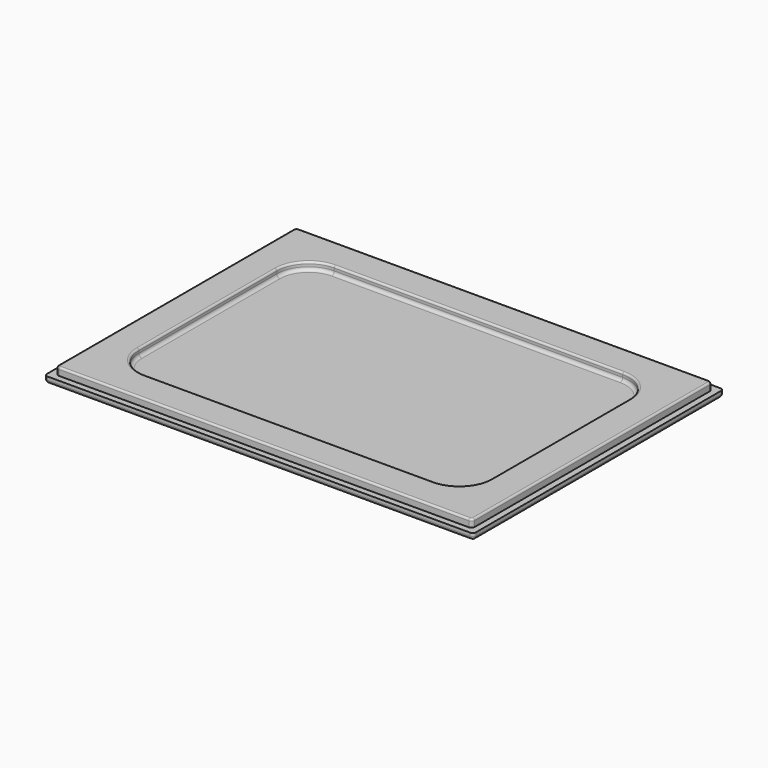
from build123d import *

# Parameters (mm, degrees)
F0_W         = 67.2
F0_H         = 49
F1_DEPTH     = 1
F2_DEPTH     = 2.2
F3_R         = 0.5
F4_R         = 0.3
F5_S2_W      = 0.5
F5_S2_H      = 0.5
F5_T3_DEPTH  = 0.5
F5_T8_ANGLE  = 90
F5_S10_W     = 0.5
F5_S10_H     = 0.5
F5_T11_DEPTH = 0.5
F5_T16_ANGLE = 90
F5_S18_W     = 0.5
F5_S18_H     = 0.5
F5_T19_DEPTH = 0.5
F5_T24_ANGLE = 90
F5_S26_W     = 0.5
F5_S26_H     = 0.5
F5_T27_DEPTH = 0.5
F5_T32_ANGLE = 90
F5_T35_DEPTH = 1.2
F5_T38_DEPTH = 1.75
F5_T41_DEPTH = 1.2
F5_T44_DEPTH = 1.75
F5_T47_DEPTH = 1.2
F5_T50_DEPTH = 1.75
F5_T53_DEPTH = 1.2
F5_T56_DEPTH = 1.75
F6_R         = 0.5


# Not quite as in the source:
# - a fillet or chamfer that OpenCascade refuses, or shapes differently, is made with other operations: its cross-section is extruded or revolved along the edge and cut away or added


with BuildPart() as f1:
    # F0 (on Top) → F1 (new body)
    with BuildSketch(Plane.XY):
        with Locations((8.3761618346, 4.5501037389)):
            Rectangle(F0_W, F0_H)
        Polygon((-24.2238381654, 20.0501037389), (-24.2238381654, 28.0501037389), (-16.2238381654, 28.0501037389), (32.9761618346, 28.0501037389), (40.9761618346, 28.0501037389), (40.9761618346, 20.0501037389), (40.9761618346, -10.9498962611), (40.9761618346, -18.9498962611), (32.9761618346, -18.9498962611), (-16.2238381654, -18.9498962611), (-24.2238381654, -18.9498962611), (-24.2238381654, -10.9498962611), align=None, mode=Mode.SUBTRACT)
        Polygon((-16.2238381654, 28.0501037389), (-24.2238381654, 28.0501037389), (-24.2238381654, 20.0501037389), (-24.2238381654, -10.9498962611), (-24.2238381654, -18.9498962611), (-16.2238381654, -18.9498962611), (32.9761618346, -18.9498962611), (40.9761618346, -18.9498962611), (40.9761618346, -10.9498962611), (40.9761618346, 20.0501037389), (40.9761618346, 28.0501037389), (32.9761618346, 28.0501037389), align=None)
        with BuildLine():
            ThreePointArc((-19.2238390446, 18.0501037389), (-17.7593729505, 21.5856376448), (-14.2238390446, 23.0501037389))
            Line((-14.2238390446, 23.0501037389), (30.9761627138, 23.0501037389))
            ThreePointArc((30.9761627138, 23.0501037389), (34.5116966197, 21.5856376448), (35.9761627138, 18.0501037389))
            Line((35.9761627138, 18.0501037389), (35.9761627138, -8.9498971403))
            ThreePointArc((35.9761627138, -8.9498971403), (34.5116966197, -12.4854310462), (30.9761627138, -13.9498971403))
            Line((30.9761627138, -13.9498971403), (-14.2238390446, -13.9498971403))
            ThreePointArc((-14.2238390446, -13.9498971403), (-17.7593729505, -12.4854310462), (-19.2238390446, -8.9498971403))
            Line((-19.2238390446, -8.9498971403), (-19.2238390446, 18.0501037389))
        make_face(mode=Mode.SUBTRACT)
        with BuildLine():
            Line((30.9761627138, 23.0501037389), (-14.2238390446, 23.0501037389))
            ThreePointArc((-14.2238390446, 23.0501037389), (-17.7593729505, 21.5856376448), (-19.2238390446, 18.0501037389))
            Line((-19.2238390446, 18.0501037389), (-19.2238390446, -8.9498971403))
            ThreePointArc((-19.2238390446, -8.9498971403), (-17.7593729505, -12.4854310462), (-14.2238390446, -13.9498971403))
            Line((-14.2238390446, -13.9498971403), (30.9761627138, -13.9498971403))
            ThreePointArc((30.9761627138, -13.9498971403), (34.5116966197, -12.4854310462), (35.9761627138, -8.9498971403))
            Line((35.9761627138, -8.9498971403), (35.9761627138, 18.0501037389))
            ThreePointArc((35.9761627138, 18.0501037389), (34.5116966197, 21.5856376448), (30.9761627138, 23.0501037389))
        make_face()
    extrude(amount=F1_DEPTH)

    # F0 (on Top) → F2 (join)
    with BuildSketch(Plane.XY):
        Polygon((-16.2238381654, 28.0501037389), (-24.2238381654, 28.0501037389), (-24.2238381654, 20.0501037389), (-24.2238381654, -10.9498962611), (-24.2238381654, -18.9498962611), (-16.2238381654, -18.9498962611), (32.9761618346, -18.9498962611), (40.9761618346, -18.9498962611), (40.9761618346, -10.9498962611), (40.9761618346, 20.0501037389), (40.9761618346, 28.0501037389), (32.9761618346, 28.0501037389), align=None)
        with BuildLine():
            ThreePointArc((-19.2238390446, 18.0501037389), (-17.7593729505, 21.5856376448), (-14.2238390446, 23.0501037389))
            Line((-14.2238390446, 23.0501037389), (30.9761627138, 23.0501037389))
            ThreePointArc((30.9761627138, 23.0501037389), (34.5116966197, 21.5856376448), (35.9761627138, 18.0501037389))
            Line((35.9761627138, 18.0501037389), (35.9761627138, -8.9498971403))
            ThreePointArc((35.9761627138, -8.9498971403), (34.5116966197, -12.4854310462), (30.9761627138, -13.9498971403))
            Line((30.9761627138, -13.9498971403), (-14.2238390446, -13.9498971403))
            ThreePointArc((-14.2238390446, -13.9498971403), (-17.7593729505, -12.4854310462), (-19.2238390446, -8.9498971403))
            Line((-19.2238390446, -8.9498971403), (-19.2238390446, 18.0501037389))
        make_face(mode=Mode.SUBTRACT)
    extrude(amount=F2_DEPTH)

    # F3
    f3_edges = [f1.edges().sort_by_distance(p)[0] for p in [
        (41.976162, 4.550104, 0),
        (8.376162, 29.050104, 0),
        (-25.223838, 4.550104, 0),
        (8.376162, -19.949896, 0),
    ]]
    fillet(f3_edges, radius=F3_R)

    # F4
    f4_edges = [f1.edges().sort_by_distance(p)[0] for p in [
        (8.376162, 28.050104, 2.2),
        (-24.223838, 4.550104, 2.2),
        (8.376162, -18.949896, 2.2),
        (40.976162, 4.550104, 2.2),
        (-19.223839, 4.550103, 2.2),
        (-17.759373, 21.585638, 2.2),
        (8.376162, 23.050104, 2.2),
        (34.511697, 21.585638, 2.2),
        (35.976163, 4.550103, 2.2),
        (34.511697, -12.485431, 2.2),
        (8.376162, -13.949897, 2.2),
        (-17.759373, -12.485431, 2.2),
    ]]
    fillet(f4_edges, radius=F4_R)

    # F5: fillet of radius 0.5 on 8 edges, made by hand


with BuildPart() as f5_tool1:
    # F5_s2 → F5_t3 (new body)
    with BuildSketch(Plane.XZ.offset(-28.5501037389)):
        with Locations((-24.9738381654, 0.25)):
            Rectangle(F5_S2_W, F5_S2_H)
    extrude(amount=-F5_T3_DEPTH)

    # F5_s4 → F5_t5 (revolve, cut)
    with BuildSketch(Plane(origin=(-24.7238381654, 28.5501037389, 0.5), x_dir=(0.7071067812, 0, 0.7071067812), z_dir=(-0.7071067812, 0, 0.7071067812))):
        with BuildLine():
            ThreePointArc((0, -0.5), (0.5, 0), (0, 0.5))
            Line((0, 0.5), (0, -0.5))
        make_face()
    revolve(axis=Axis((-24.7238381654, 28.5501037389, 0.5), (0, 1, 0)), mode=Mode.SUBTRACT)


with BuildPart() as f5_tool6:
    # F5_s7 → F5_t8 (revolve)
    with BuildSketch(Plane.YZ.offset(-23.7238381654)):
        with BuildLine():
            ThreePointArc((27.7501037389, 2.2), (27.9622357733, 2.1121320344), (28.0501037389, 1.9))
            Line((28.0501037389, 1.9), (28.0501037389, 2.2))
            Line((28.0501037389, 2.2), (27.7501037389, 2.2))
        make_face()
    revolve(axis=Axis((-23.7238381654, 27.5501037389, 2.2), (0, 0, 1)), revolution_arc=F5_T8_ANGLE)


with BuildPart() as f5_tool9:
    # F5_s10 → F5_t11 (new body)
    with BuildSketch(Plane.XZ.offset(19.4498962611)):
        with Locations((-24.9738381654, 0.25)):
            Rectangle(F5_S10_W, F5_S10_H)
    extrude(amount=F5_T11_DEPTH)

    # F5_s12 → F5_t13 (revolve, cut)
    with BuildSketch(Plane(origin=(-24.7238381654, -19.4498962611, 0.5), x_dir=(0.7071067812, 0, 0.7071067812), z_dir=(0.7071067812, 0, -0.7071067812))):
        with BuildLine():
            ThreePointArc((0, -0.5), (0.5, 0), (0, 0.5))
            Line((0, 0.5), (0, -0.5))
        make_face()
    revolve(axis=Axis((-24.7238381654, -19.4498962611, 0.5), (0, -1, 0)), mode=Mode.SUBTRACT)


with BuildPart() as f5_tool14:
    # F5_s15 → F5_t16 (revolve)
    with BuildSketch(Plane.XZ.offset(18.4498962611)):
        with BuildLine():
            ThreePointArc((-23.9238381654, 2.2), (-24.1359701998, 2.1121320344), (-24.2238381654, 1.9))
            Line((-24.2238381654, 1.9), (-24.2238381654, 2.2))
            Line((-24.2238381654, 2.2), (-23.9238381654, 2.2))
        make_face()
    revolve(axis=Axis((-23.7238381654, -18.4498962611, 2.2), (0, 0, 1)), revolution_arc=F5_T16_ANGLE)


with BuildPart() as f5_tool17:
    # F5_s18 → F5_t19 (new body)
    with BuildSketch(Plane.YZ.offset(41.4761618346)):
        with Locations((-19.6998962611, 0.25)):
            Rectangle(F5_S18_W, F5_S18_H)
    extrude(amount=F5_T19_DEPTH)

    # F5_s20 → F5_t21 (revolve, cut)
    with BuildSketch(Plane(origin=(41.4761618346, -19.4498962611, 0.5), x_dir=(0, 0.7071067812, 0.7071067812), z_dir=(0, 0.7071067812, -0.7071067812))):
        with BuildLine():
            ThreePointArc((0, -0.5), (0.5, 0), (0, 0.5))
            Line((0, 0.5), (0, -0.5))
        make_face()
    revolve(axis=Axis((41.4761618346, -19.4498962611, 0.5), (1, 0, 0)), mode=Mode.SUBTRACT)


with BuildPart() as f5_tool22:
    # F5_s23 → F5_t24 (revolve)
    with BuildSketch(Plane.YZ.offset(40.4761618346)):
        with BuildLine():
            ThreePointArc((-18.6498962611, 2.2), (-18.8620282955, 2.1121320344), (-18.9498962611, 1.9))
            Line((-18.9498962611, 1.9), (-18.9498962611, 2.2))
            Line((-18.9498962611, 2.2), (-18.6498962611, 2.2))
        make_face()
    revolve(axis=Axis((40.4761618346, -18.4498962611, 2.2), (0, 0, 1)), revolution_arc=F5_T24_ANGLE)


with BuildPart() as f5_tool25:
    # F5_s26 → F5_t27 (new body)
    with BuildSketch(Plane.YZ.offset(41.4761618346)):
        with Locations((28.8001037389, 0.25)):
            Rectangle(F5_S26_W, F5_S26_H)
    extrude(amount=F5_T27_DEPTH)

    # F5_s28 → F5_t29 (revolve, cut)
    with BuildSketch(Plane(origin=(41.4761618346, 28.5501037389, 0.5), x_dir=(0, -0.7071067812, 0.7071067812), z_dir=(0, 0.7071067812, 0.7071067812))):
        with BuildLine():
            ThreePointArc((0, -0.5), (0.5, 0), (0, 0.5))
            Line((0, 0.5), (0, -0.5))
        make_face()
    revolve(axis=Axis((41.4761618346, 28.5501037389, 0.5), (1, 0, 0)), mode=Mode.SUBTRACT)


with BuildPart() as f5_tool30:
    # F5_s31 → F5_t32 (revolve)
    with BuildSketch(Plane.XZ.offset(-27.5501037389)):
        with BuildLine():
            ThreePointArc((40.6761618346, 2.2), (40.888293869, 2.1121320344), (40.9761618346, 1.9))
            Line((40.9761618346, 1.9), (40.9761618346, 2.2))
            Line((40.9761618346, 2.2), (40.6761618346, 2.2))
        make_face()
    revolve(axis=Axis((40.4761618346, 27.5501037389, 2.2), (0, 0, 1)), revolution_arc=F5_T32_ANGLE)


with BuildPart() as f5_tool33:
    # F5_s34 → F5_t35 (new body)
    with BuildSketch(Plane.XY.offset(1)):
        with BuildLine():
            ThreePointArc((40.4761618346, 28.0501037389), (40.8297152252, 27.9036571295), (40.9761618346, 27.5501037389))
            Line((40.9761618346, 27.5501037389), (40.9761618346, 28.0501037389))
            Line((40.9761618346, 28.0501037389), (40.4761618346, 28.0501037389))
        make_face()
    extrude(amount=F5_T35_DEPTH)


with BuildPart() as f5_tool36:
    # F5_s37 → F5_t38 (new body)
    with BuildSketch(Plane.XY.offset(0.5)):
        with BuildLine():
            ThreePointArc((41.9761618346, 28.5501037389), (41.8297152252, 28.9036571295), (41.4761618346, 29.0501037389))
            Line((41.4761618346, 29.0501037389), (41.9761618346, 29.0501037389))
            Line((41.9761618346, 29.0501037389), (41.9761618346, 28.5501037389))
        make_face()
    extrude(amount=F5_T38_DEPTH)


with BuildPart() as f5_tool39:
    # F5_s40 → F5_t41 (new body)
    with BuildSketch(Plane.XY.offset(1)):
        with BuildLine():
            ThreePointArc((40.4761618346, -18.9498962611), (40.8297152252, -18.8034496517), (40.9761618346, -18.4498962611))
            Line((40.9761618346, -18.4498962611), (40.9761618346, -18.9498962611))
            Line((40.9761618346, -18.9498962611), (40.4761618346, -18.9498962611))
        make_face()
    extrude(amount=F5_T41_DEPTH)


with BuildPart() as f5_tool42:
    # F5_s43 → F5_t44 (new body)
    with BuildSketch(Plane.XY.offset(0.5)):
        with BuildLine():
            ThreePointArc((41.9761618346, -19.4498962611), (41.8297152252, -19.8034496517), (41.4761618346, -19.9498962611))
            Line((41.4761618346, -19.9498962611), (41.9761618346, -19.9498962611))
            Line((41.9761618346, -19.9498962611), (41.9761618346, -19.4498962611))
        make_face()
    extrude(amount=F5_T44_DEPTH)


with BuildPart() as f5_tool45:
    # F5_s46 → F5_t47 (new body)
    with BuildSketch(Plane.XY.offset(1)):
        with BuildLine():
            ThreePointArc((-24.2238381654, -18.4498962611), (-24.077391556, -18.8034496517), (-23.7238381654, -18.9498962611))
            Line((-23.7238381654, -18.9498962611), (-24.2238381654, -18.9498962611))
            Line((-24.2238381654, -18.9498962611), (-24.2238381654, -18.4498962611))
        make_face()
    extrude(amount=F5_T47_DEPTH)


with BuildPart() as f5_tool48:
    # F5_s49 → F5_t50 (new body)
    with BuildSketch(Plane.XY.offset(0.5)):
        with BuildLine():
            ThreePointArc((-24.7238381654, -19.9498962611), (-25.077391556, -19.8034496517), (-25.2238381654, -19.4498962611))
            Line((-25.2238381654, -19.4498962611), (-25.2238381654, -19.9498962611))
            Line((-25.2238381654, -19.9498962611), (-24.7238381654, -19.9498962611))
        make_face()
    extrude(amount=F5_T50_DEPTH)


with BuildPart() as f5_tool51:
    # F5_s52 → F5_t53 (new body)
    with BuildSketch(Plane.XY.offset(1)):
        with BuildLine():
            ThreePointArc((-24.2238381654, 27.5501037389), (-24.077391556, 27.9036571295), (-23.7238381654, 28.0501037389))
            Line((-23.7238381654, 28.0501037389), (-24.2238381654, 28.0501037389))
            Line((-24.2238381654, 28.0501037389), (-24.2238381654, 27.5501037389))
        make_face()
    extrude(amount=F5_T53_DEPTH)


with BuildPart() as f5_tool54:
    # F5_s55 → F5_t56 (new body)
    with BuildSketch(Plane.XY.offset(0.5)):
        with BuildLine():
            ThreePointArc((-24.7238381654, 29.0501037389), (-25.077391556, 28.9036571295), (-25.2238381654, 28.5501037389))
            Line((-25.2238381654, 28.5501037389), (-25.2238381654, 29.0501037389))
            Line((-25.2238381654, 29.0501037389), (-24.7238381654, 29.0501037389))
        make_face()
    extrude(amount=F5_T56_DEPTH)


with BuildPart() as f1_1:
    add(f1.part)

    # F5_t57: cut F5_tool1, F5_tool6, F5_tool9, F5_tool14, F5_tool17, F5_tool22, F5_tool25, F5_tool30, F5_tool33, F5_tool36, F5_tool39, F5_tool42, F5_tool45, F5_tool48, F5_tool51, F5_tool54
    add([f5_tool1.part, f5_tool6.part, f5_tool9.part, f5_tool14.part, f5_tool17.part, f5_tool22.part, f5_tool25.part, f5_tool30.part, f5_tool33.part, f5_tool36.part, f5_tool39.part, f5_tool42.part, f5_tool45.part, f5_tool48.part, f5_tool51.part, f5_tool54.part], mode=Mode.SUBTRACT)

    # F6
    f6_edges = [f1_1.edges().sort_by_distance(p)[0] for p in [
        (-17.759373, -12.485431, 1),
        (-19.223839, 4.550103, 1),
        (-17.759373, 21.585638, 1),
        (8.376162, 23.050104, 1),
        (34.511697, 21.585638, 1),
        (35.976163, 4.550103, 1),
        (34.511697, -12.485431, 1),
        (8.376162, -13.949897, 1),
    ]]
    fillet(f6_edges, radius=F6_R)


solid = f1_1.part
